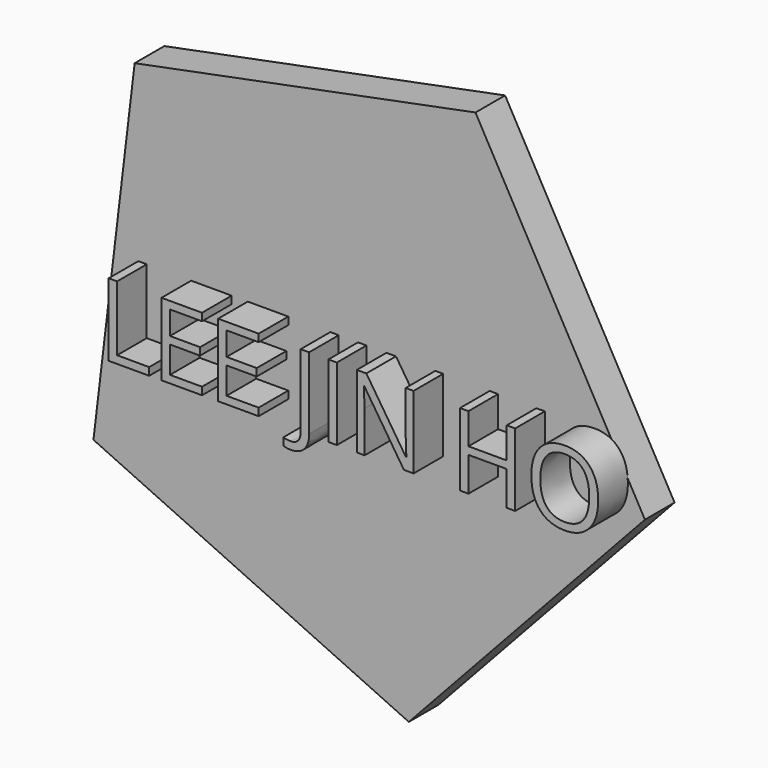
from build123d import *

# Parameters (mm, degrees)
F1_DEPTH     = 7
F2_TEXT_SIZE = 19.2506781448
F3_DEPTH     = 7


# Not quite as in the source:
# - Text() gives the source's letters only with a copy of the font that has no kerning and outlines rounded to 1/6400 em; it was checked with that copy


with BuildPart() as f1:
    # F0 (on Front) → F1 (new body)
    with BuildSketch(Plane.XZ):
        Polygon((55.483352482, -6.6271556232), (23.4480983618, 50.719900212), (-40.9916307229, 37.9737778602), (-48.7823194028, -27.2508148132), (10.8424992819, -54.8157076359), align=None)
    extrude(amount=F1_DEPTH)

    # F2 (on face) → F3 (join)
    with BuildSketch(Plane.XZ.offset(7)):
        with Locations((-42.194634676, -8.4990067407)):
            Text('LEE JIN HO', F2_TEXT_SIZE, font='Open Sans', text_align=(TextAlign.LEFT, TextAlign.BOTTOM))
    extrude(amount=F3_DEPTH)


solid = f1.part
